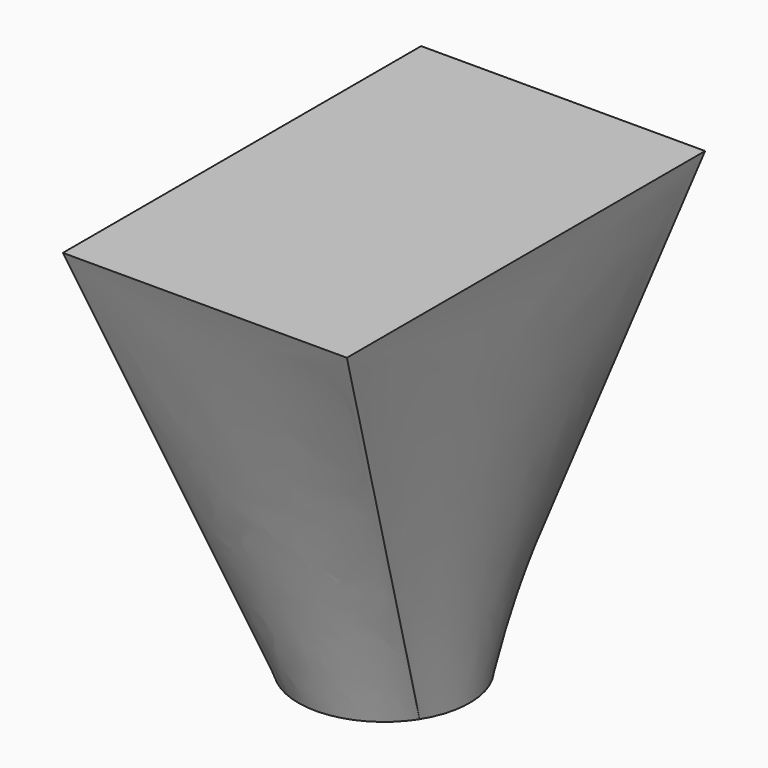
from build123d import *

# Parameters (mm, degrees)
F2_W = 87.2814878821
F2_H = 137.6141756773


# Not quite as in the source:
# - the arcs of a loft's sections are written as splines that run evenly, so that the points pair up as in the source's solid


with BuildPart() as f3:
    # F2 (on offset) → F3 section 0
    with BuildSketch(Plane.XY.offset(127)):
        Rectangle(F2_W, F2_H)
    # F1 (on Top) → F3 section 1
    with BuildSketch(Plane.XY):
        with BuildLine():
            add(Edge.make_bspline(
                [(14.0971746488, 22.2266040112), (12.642446818, 23.1492619344), (11.0968833316, 23.9286224004), (7.8833287822, 25.1708743783), (6.2154171805, 25.6337351731), (2.8212588422, 26.2251842358), (1.0950960328, 26.3537578788), (-2.3492304928, 26.2716749703), (-4.0673090413, 26.0610204485), (-7.4294402175, 25.3085599691), (-9.0734097099, 24.7667726176), (-12.2241407211, 23.3728512015), (-13.7308243318, 22.5207516043), (-16.5490743521, 20.5389368698), (-17.860571075, 19.4092707367), (-20.2380363367, 16.9157227126), (-21.303946088, 15.5519024795), (-22.2266040112, 14.0971746488)],
                knots=[0, 0, 0, 0, 0.125, 0.125, 0.25, 0.25, 0.375, 0.375, 0.5, 0.5, 0.625, 0.625, 0.75, 0.75, 0.875, 0.875, 1, 1, 1, 1], degree=3))
            add(Edge.make_bspline(
                [(-22.2266040112, 14.0971746488), (-23.1492619344, 12.642446818), (-23.9286224004, 11.0968833316), (-25.1708743783, 7.8833287822), (-25.6337351731, 6.2154171805), (-26.2251842358, 2.8212588422), (-26.3537578788, 1.0950960328), (-26.2716749703, -2.3492304928), (-26.0610204485, -4.0673090413), (-25.3085599691, -7.4294402175), (-24.7667726176, -9.0734097099), (-23.3728512015, -12.2241407211), (-22.5207516043, -13.7308243318), (-20.5389368698, -16.5490743521), (-19.4092707367, -17.860571075), (-16.9157227126, -20.2380363367), (-15.5519024795, -21.303946088), (-14.0971746488, -22.2266040112)],
                knots=[0, 0, 0, 0, 0.125, 0.125, 0.25, 0.25, 0.375, 0.375, 0.5, 0.5, 0.625, 0.625, 0.75, 0.75, 0.875, 0.875, 1, 1, 1, 1], degree=3))
            add(Edge.make_bspline(
                [(-14.0971746488, -22.2266040112), (-12.642446818, -23.1492619344), (-11.0968833316, -23.9286224004), (-7.8833287822, -25.1708743783), (-6.2154171805, -25.6337351731), (-2.8212588422, -26.2251842358), (-1.0950960328, -26.3537578788), (2.3492304928, -26.2716749703), (4.0673090413, -26.0610204485), (7.4294402175, -25.3085599691), (9.0734097099, -24.7667726176), (12.2241407211, -23.3728512015), (13.7308243318, -22.5207516043), (16.5490743521, -20.5389368698), (17.860571075, -19.4092707367), (20.2380363367, -16.9157227126), (21.303946088, -15.5519024795), (22.2266040112, -14.0971746488)],
                knots=[0, 0, 0, 0, 0.125, 0.125, 0.25, 0.25, 0.375, 0.375, 0.5, 0.5, 0.625, 0.625, 0.75, 0.75, 0.875, 0.875, 1, 1, 1, 1], degree=3))
            add(Edge.make_bspline(
                [(22.2266040112, -14.0971746488), (23.1492619344, -12.642446818), (23.9286224004, -11.0968833316), (25.1708743783, -7.8833287822), (25.6337351731, -6.2154171805), (26.2251842358, -2.8212588422), (26.3537578788, -1.0950960328), (26.2716749703, 2.3492304928), (26.0610204485, 4.0673090413), (25.3085599691, 7.4294402175), (24.7667726176, 9.0734097099), (23.3728512015, 12.2241407211), (22.5207516043, 13.7308243318), (20.5389368698, 16.5490743521), (19.4092707367, 17.860571075), (16.9157227126, 20.2380363367), (15.5519024795, 21.303946088), (14.0971746488, 22.2266040112)],
                knots=[0, 0, 0, 0, 0.125, 0.125, 0.25, 0.25, 0.375, 0.375, 0.5, 0.5, 0.625, 0.625, 0.75, 0.75, 0.875, 0.875, 1, 1, 1, 1], degree=3))
        make_face()
    loft(ruled=True)


solid = f3.part
